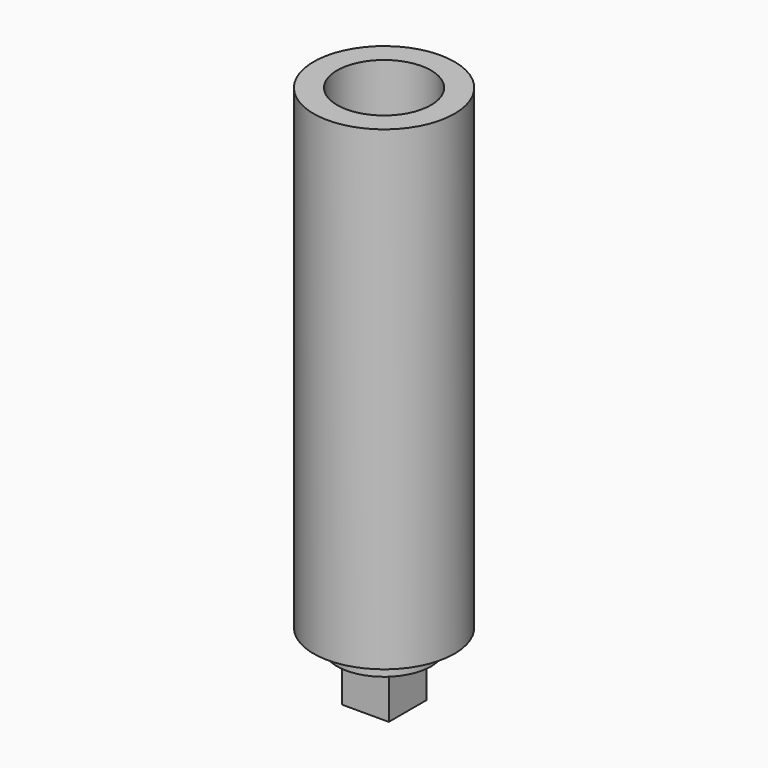
from build123d import *

# Parameters (mm, degrees)
F0_R          = 9.525
F0_R_2        = 6.35
F1_DEPTH      = 64.262
F2_R          = 6.35
F3_DEPTH      = 63.5
F4_DEPTH      = 19.05
F4_DEPTH_BACK = 2.54
F5_W          = 6.35
F5_H          = 6.35
F6_DEPTH      = 6.35


with BuildPart() as f1:
    # F0 (on Top) → F1 (new body)
    with BuildSketch(Plane.XY):
        Circle(F0_R)
        Circle(F0_R_2, mode=Mode.SUBTRACT)
    extrude(amount=F1_DEPTH)

    # F2 (on face) → F3 (cut)
    with BuildSketch(Plane.XY.offset(64.262)):
        Circle(F2_R)
    extrude(amount=-F3_DEPTH, mode=Mode.SUBTRACT)


with BuildPart() as f4:
    # F0 (on Top) → F4 (new body, two sides)
    with BuildSketch(Plane.XY) as f4_sk:
        Circle(F0_R_2)
    extrude(amount=F4_DEPTH)
    extrude(f4_sk.sketch, amount=-F4_DEPTH_BACK)


with BuildPart() as f6:
    # F5 (on face) → F6 (new body)
    with BuildSketch(Plane(origin=(0, 0, -2.54), x_dir=(1, 0, 0), z_dir=(0, 0, -1))):
        Rectangle(F5_W, F5_H)
    extrude(amount=F6_DEPTH)


solid = Compound([f1.part, f4.part, f6.part])
